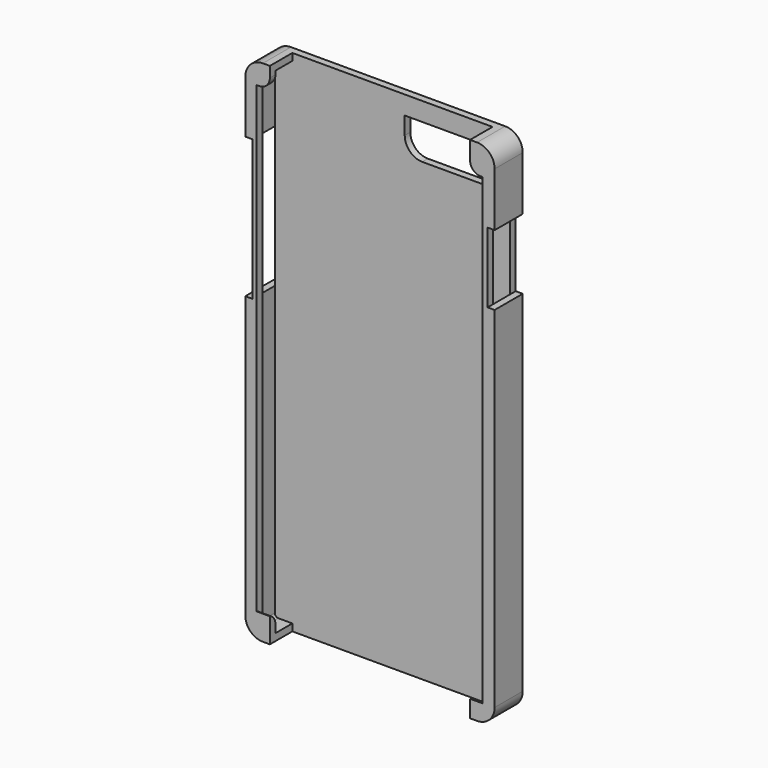
from build123d import *

# Parameters (mm, degrees)
F0_W         = 71
F0_H         = 145
F1_DEPTH     = 2
F2_W         = 7
F2_H         = 145
F3_DEPTH     = 8
F4_T         = 2
F5_W         = 3.7458891392
F5_H         = 131.9372802973
F6_DEPTH     = 2
F7_W         = 3.5460759103
F7_H         = 131.9372802973
F8_DEPTH     = 2
F9_R         = 5
F11_DEPTH    = 2.5
F13_DEPTH    = 2
F15_T1_DEPTH = 9.5
F15_T3_DEPTH = 10.6171437222
F15_T5_DEPTH = 10.816956951
F16_R        = 1
F14_W        = 10
F14_H        = 20
F17_DEPTH    = 2


# Not quite as in the source:
# - a fillet or chamfer that OpenCascade refuses, or shapes differently, is made with other operations: its cross-section is extruded or revolved along the edge and cut away or added
# - a shell that OpenCascade refuses in one call is made with other operations: the cavity is built on its own and cut out
# - a feature names something its author has since deleted; it is built from what else it names


with BuildPart() as f1:
    # F0 (on Front) → F1 (new body)
    with BuildSketch(Plane.XZ):
        Rectangle(F0_W, F0_H)
    extrude(amount=F1_DEPTH)

    # F2 (on face) → F3 (join)
    with BuildSketch(Plane.XZ.offset(2)):
        with Locations((-32, 0)):
            Rectangle(F2_W, F2_H)
        with Locations((32, 0)):
            Rectangle(F2_W, F2_H)
    extrude(amount=F3_DEPTH)

    # F4: shell of thickness 2, made by hand


with BuildPart() as f4_core1:
    # F4_t2: copy of F1
    add(f1.part)

    # the walls: a layer under each face that stays
    f4_faces = [f4_core1.faces().sort_by_distance(p)[0] for p in [
        (23.6666666667, -1.6666666667, 72.5),
        (0, 0, 0),
        (-23.6666666667, -1.6666666667, -72.5),
        (-35.5, -5, 0),
        (-32, -10, 0),
        (0, -2, 0),
        (32, -10, 0),
        (35.5, -5, 0),
    ]]
    thicken(f4_faces, amount=-F4_T, mode=Mode.SUBTRACT)


with BuildPart() as f1_1:
    add(f1.part)

    # what is left inside the walls is the cavity
    f4_cavity = [f4_core1.part.solids().sort_by_distance(p)[0] for p in [
        (33.48, -6, 0),
        (-28.52, -6, 0),
    ]]
    add(f4_cavity, mode=Mode.SUBTRACT)

    # F5 (on face) → F6 (cut)
    with BuildSketch(Plane.XZ.offset(10)):
        with Locations((-30.3729445696, 0.5088895559)):
            Rectangle(F5_W, F5_H)
    extrude(amount=-F6_DEPTH, mode=Mode.SUBTRACT)

    # F7 (on face) → F8 (cut)
    with BuildSketch(Plane.XZ.offset(10)):
        with Locations((30.2730379552, -1.6313598514)):
            Rectangle(F7_W, F7_H)
    extrude(amount=-F8_DEPTH, mode=Mode.SUBTRACT)

    # F9
    f9_edges = [f1_1.edges().sort_by_distance(p)[0] for p in [
        (-35.5, -5, 72.5),
        (35.5, -5, 72.5),
        (35.5, -5, -72.5),
        (-35.5, -5, -72.5),
    ]]
    fillet(f9_edges, radius=F9_R)

    # F10 (on face) → F11 (cut)
    with BuildSketch(Plane.XZ.offset(2)):
        with BuildLine():
            ThreePointArc((28.5, 62.2240006924), (27.0355339059, 65.7595345983), (23.5, 67.2240006924))
            Line((23.5, 67.2240006924), (3.5, 67.2240006924))
            Line((3.5, 67.2240006924), (3.5, 62.2240006924))
            ThreePointArc((3.5, 62.2240006924), (4.9644660941, 58.6884667864), (8.5, 57.2240006924))
            Line((8.5, 57.2240006924), (28.5, 57.2240006924))
            Line((28.5, 57.2240006924), (28.5, 62.2240006924))
        make_face()
    extrude(amount=-F11_DEPTH, mode=Mode.SUBTRACT)

    # F12 (on face) → F13 (cut)
    with BuildSketch(Plane(origin=(-35.5, 0, 0), x_dir=(0, -1, 0), z_dir=(-1, 0, 0))):
        Polygon((10, 52.5), (0, 52.5), (0, 12.5), (10, 12.5), (10, 47.0733729486), align=None)
    extrude(amount=-F13_DEPTH, mode=Mode.SUBTRACT)

    # F15: fillet of radius 3 on 4 edges, made by hand

    # F15_s2 → F15_t1 (cut)
    with BuildSketch(Plane.XZ.offset(8)):
        with BuildLine():
            ThreePointArc((28.5, 67.3372802973), (29.3786796564, 65.2159599537), (31.5, 64.3372802973))
            Line((31.5, 64.3372802973), (28.5, 64.3372802973))
            Line((28.5, 64.3372802973), (28.5, 67.3372802973))
        make_face()
        with BuildLine():
            ThreePointArc((-28.5, 69.4775297046), (-29.3786796564, 67.356209361), (-31.5, 66.4775297046))
            Line((-31.5, 66.4775297046), (-28.5, 66.4775297046))
            Line((-28.5, 66.4775297046), (-28.5, 69.4775297046))
        make_face()
    extrude(amount=F15_T1_DEPTH, mode=Mode.SUBTRACT)

    # F15_s4 → F15_t3 (cut)
    with BuildSketch(Plane.YZ.offset(21.4289321881)):
        with BuildLine():
            ThreePointArc((-10, -67.6), (-8.5505102572, -68.6963763172), (-8, -70.4284271247))
            Line((-8, -70.4284271247), (-8, -67.6))
            Line((-8, -67.6), (-10, -67.6))
        make_face()
    extrude(amount=F15_T3_DEPTH, mode=Mode.SUBTRACT)

    # F15_s6 → F15_t5 (cut)
    with BuildSketch(Plane.YZ.offset(-32.2458891392)):
        with BuildLine():
            ThreePointArc((-8, -68.2881777175), (-8.5505102572, -66.5561269099), (-10, -65.4597505927))
            Line((-10, -65.4597505927), (-8, -65.4597505927))
            Line((-8, -65.4597505927), (-8, -68.2881777175))
        make_face()
    extrude(amount=F15_T5_DEPTH, mode=Mode.SUBTRACT)

    # F16
    f16_edges = [f1_1.edges().sort_by_distance(p)[0] for p in [
        (33.5, -5, 70.5),
        (-33.5, -5, 70.5),
        (-33.5, -5, -70.5),
        (33.5, -5, -70.5),
    ]]
    fillet(f16_edges, radius=F16_R)

    # F14 (on face) → F17 (cut)
    with BuildSketch(Plane.YZ.offset(35.5)):
        with Locations((-5, 42.1337091768)):
            Rectangle(F14_W, F14_H)
    extrude(amount=-F17_DEPTH, mode=Mode.SUBTRACT)


solid = f1_1.part
